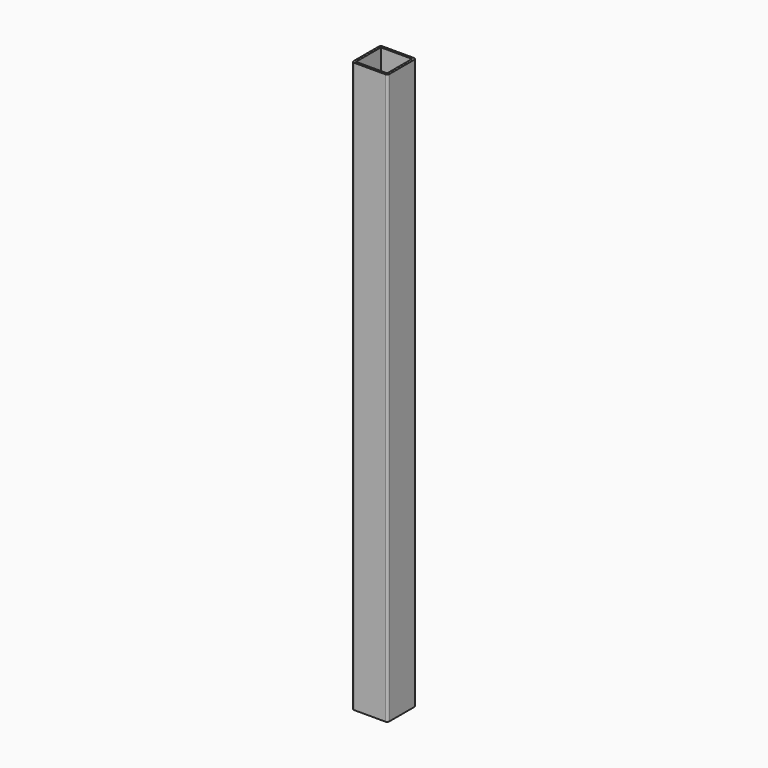
from build123d import *

# Parameters (mm, degrees)
F1_DEPTH = 812.8
F2_T     = 3.175


# Not quite as in the source:
# - a shell that OpenCascade refuses in one call is made with other operations: the cavity is built on its own and cut out


with BuildPart() as f1:
    # F0 (on Top) → F1 (new body)
    with BuildSketch(Plane.XY):
        with BuildLine():
            Line((22.225, 25.4), (-22.225, 25.4))
            ThreePointArc((-22.225, 25.4), (-24.4700640303, 24.4700640303), (-25.4, 22.225))
            Line((-25.4, 22.225), (-25.4, -22.225))
            ThreePointArc((-25.4, -22.225), (-24.4700640303, -24.4700640303), (-22.225, -25.4))
            Line((-22.225, -25.4), (22.225, -25.4))
            ThreePointArc((22.225, -25.4), (24.4700640303, -24.4700640303), (25.4, -22.225))
            Line((25.4, -22.225), (25.4, 22.225))
            ThreePointArc((25.4, 22.225), (24.4700640303, 24.4700640303), (22.225, 25.4))
        make_face()
    extrude(amount=F1_DEPTH)

    # F2: shell of thickness 3.175, made by hand


with BuildPart() as f2_core1:
    # F2_t2: copy of F1
    add(f1.part)

    # the walls: a layer under each face that stays
    f2_faces = [f2_core1.faces().sort_by_distance(p)[0] for p in [
        (0, 25.4, 406.4),
        (-25.4, 0, 406.4),
        (0, -25.4, 406.4),
        (25.4, 0, 406.4),
        (0, 0, 0),
    ]]
    thicken(f2_faces, amount=-F2_T, mode=Mode.SUBTRACT)


with BuildPart() as f1_1:
    add(f1.part)

    # what is left inside the walls is the cavity
    f2_cavity = [f2_core1.part.solids().sort_by_distance(p)[0] for p in [
        (0, 22.19325, 542.925),
    ]]
    add(f2_cavity, mode=Mode.SUBTRACT)


solid = f1_1.part
